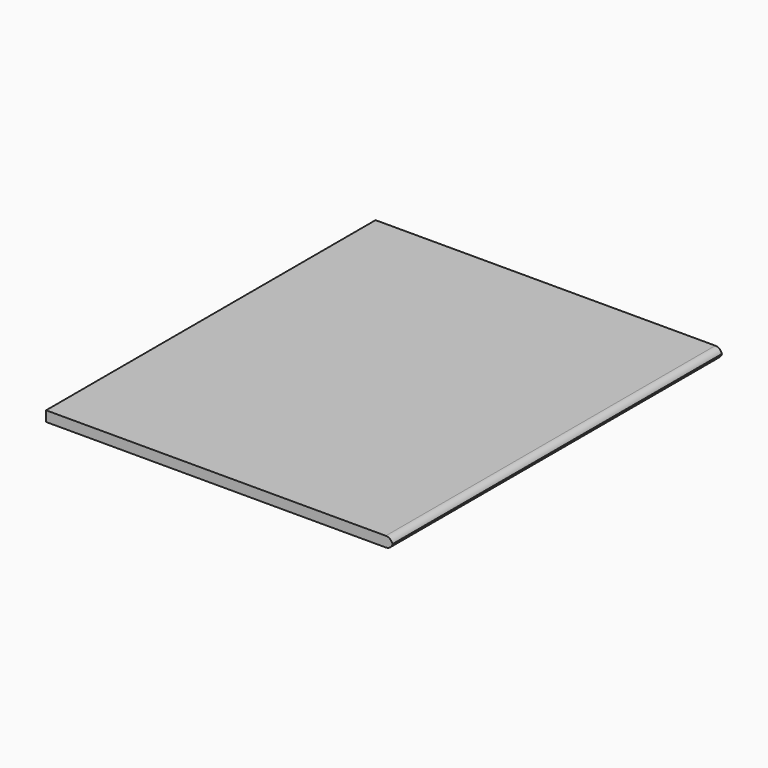
from build123d import *

# Parameters (mm, degrees)
F0_W        = 641.35
F0_H        = 762
F1_DEPTH    = 19.05
F2_T1_DEPTH = 825.5


# Not quite as in the source:
# - a fillet or chamfer that OpenCascade refuses, or shapes differently, is made with other operations: its cross-section is extruded or revolved along the edge and cut away or added


with BuildPart() as f1:
    # F0 (on Top) → F1 (new body)
    with BuildSketch(Plane.XY):
        Rectangle(F0_W, F0_H)
    extrude(amount=F1_DEPTH)

    # F2: fillet of radius 12.7 on 2 edges, made by hand

    # F2_s2 → F2_t1 (cut)
    with BuildSketch(Plane.XZ.offset(-412.75)):
        with BuildLine():
            ThreePointArc((320.675, 6.35), (316.9552561211, 15.3302561211), (307.975, 19.05))
            Line((307.975, 19.05), (320.675, 19.05))
            Line((320.675, 19.05), (320.675, 6.35))
        make_face()
        with BuildLine():
            ThreePointArc((320.675, 12.7), (316.9552561211, 3.7197438789), (307.975, 0))
            Line((307.975, 0), (320.675, 0))
            Line((320.675, 0), (320.675, 12.7))
        make_face()
    extrude(amount=F2_T1_DEPTH, mode=Mode.SUBTRACT)


solid = f1.part
